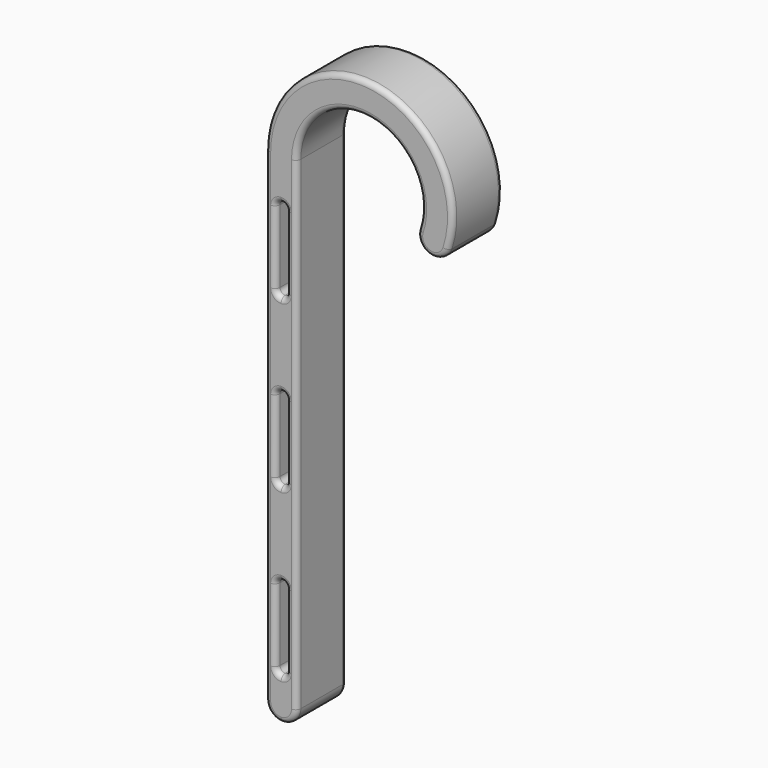
from build123d import *

# Parameters (mm, degrees)
F0_W     = 3.175
F0_H     = 25.4
F1_DEPTH = 19.05
F2_R     = 4.76249
F3_F1_R  = 1.5874
F3_F2_R  = 1.5875
F4_R     = 1.58749


# Not quite as in the source:
# - a fillet or chamfer is up to 0.001 mm smaller than in the source, because OpenCascade refuses the exact size
# - a feature names something its author has since deleted; it is built from what else it names


with BuildPart() as f1:
    # F0 (on Front) → F1 (new body)
    with BuildSketch(Plane.XZ):
        with BuildLine():
            ThreePointArc((17.145, 0), (-11.43, 28.575), (-40.005, 0))
            Line((-40.005, 0), (-40.005, -152.4))
            Line((-40.005, -152.4), (-30.48, -152.4))
            Line((-30.48, -152.4), (-30.48, 0))
            ThreePointArc((-30.48, 0), (-6.4994971908, 18.4008869908), (5.0677839421, -9.525))
            Line((5.0677839421, -9.525), (13.3166759131, -14.2875))
            ThreePointArc((13.3166759131, -14.2875), (16.1713304862, -7.3957542138), (17.145, 0))
        make_face()
        with Locations((-35.2425, -127)):
            Rectangle(F0_W, F0_H, mode=Mode.SUBTRACT)
        with Locations((-35.2425, -76.2)):
            Rectangle(F0_W, F0_H, mode=Mode.SUBTRACT)
        with Locations((-35.2425, -25.4)):
            Rectangle(F0_W, F0_H, mode=Mode.SUBTRACT)
    extrude(amount=F1_DEPTH)

    # F2 (radius 4.7625 in the source; OpenCascade refuses exactly that, so slightly less here)
    f2_edges = [f1.edges().sort_by_distance(p)[0] for p in [
        (13.316676, -9.525, -14.2875),
        (5.067784, -9.525, -9.525),
        (-30.48, -9.525, -152.4),
        (-40.005, -9.525, -152.4),
    ]]
    fillet(f2_edges, radius=F2_R)

    # F3: fillet of radius 1.5875 on 24 edges, made by hand

    # F3_f1 (radius 1.5875 in the source; OpenCascade refuses exactly that, so slightly less here)
    f3_f1_edges = [f1.edges().sort_by_distance(p)[0] for p in [
        (-36.83, -9.525, -12.7),
        (-33.655, -9.525, -12.7),
        (-36.83, -9.525, -63.5),
        (-33.655, -9.525, -63.5),
        (-36.83, -9.525, -114.3),
        (-33.655, -9.525, -114.3),
        (-33.655, -9.525, -139.7),
        (-36.83, -9.525, -139.7),
        (-33.655, -9.525, -88.9),
        (-36.83, -9.525, -88.9),
        (-33.655, -9.525, -38.1),
        (-36.83, -9.525, -38.1),
    ]]
    fillet(f3_f1_edges, radius=F3_F1_R)

    # F3_f2
    f3_f2_edges = [f1.edges().sort_by_distance(p)[0] for p in [
        (-35.2425, 0, -12.7),
        (-35.2425, -19.05, -12.7),
        (-35.2425, 0, -63.5),
        (-35.2425, -19.05, -63.5),
        (-35.2425, 0, -114.3),
        (-35.2425, -19.05, -114.3),
        (-35.2425, 0, -139.7),
        (-35.2425, -19.05, -139.7),
        (-35.2425, 0, -88.9),
        (-35.2425, -19.05, -88.9),
        (-35.2425, 0, -38.1),
        (-35.2425, -19.05, -38.1),
        (-34.1199386955, -19.05, -37.6350613045),
        (-36.3650613045, -19.05, -37.6350613045),
        (-34.1199386955, 0, -37.6350613045),
        (-36.3650613045, 0, -37.6350613045),
        (-34.1199386955, -19.05, -88.4350613045),
        (-36.3650613045, -19.05, -88.4350613045),
        (-34.1199386955, 0, -88.4350613045),
        (-36.3650613045, 0, -88.4350613045),
        (-34.1199386955, -19.05, -139.2350613045),
        (-36.3650613045, -19.05, -139.2350613045),
        (-34.1199386955, 0, -139.2350613045),
        (-36.3650613045, 0, -139.2350613045),
        (-36.3650613045, -19.05, -114.7649386955),
        (-34.1199386955, -19.05, -114.7649386955),
        (-36.3650613045, 0, -114.7649386955),
        (-34.1199386955, 0, -114.7649386955),
        (-36.3650613045, -19.05, -63.9649386955),
        (-34.1199386955, -19.05, -63.9649386955),
        (-36.3650613045, 0, -63.9649386955),
        (-34.1199386955, 0, -63.9649386955),
        (-36.3650613045, -19.05, -13.1649386955),
        (-34.1199386955, -19.05, -13.1649386955),
        (-36.3650613045, 0, -13.1649386955),
        (-34.1199386955, 0, -13.1649386955),
    ]]
    fillet(f3_f2_edges, radius=F3_F2_R)

    # F4 (radius 1.5875 in the source; OpenCascade refuses exactly that, so slightly less here)
    f4_edges = [f1.edges().sort_by_distance(p)[0] for p in [
        (-35.2425, -19.05, -11.1125),
        (-37.487593, -19.05, -12.042407),
        (-32.997407, -19.05, -12.042407),
        (-38.4175, -19.05, -25.4),
        (-32.0675, -19.05, -25.4),
        (-37.487593, -19.05, -38.757593),
        (-32.997407, -19.05, -38.757593),
        (-35.2425, -19.05, -39.6875),
        (-6.845871, -19.05, 28.2049),
        (12.845575, -19.05, -11.994292),
        (-40.005, -19.05, -73.818755),
        (8.775578, -19.05, -11.665696),
        (-38.610099, -19.05, -151.005099),
        (6.703786, -19.05, -9.229997),
        (-35.2425, -19.05, -152.4),
        (-8.373915, -19.05, 18.803267),
        (-31.874901, -19.05, -151.005099),
        (-30.48, -19.05, -73.818755),
        (-35.2425, -19.05, -61.9125),
        (-37.487593, -19.05, -62.842407),
        (-32.997407, -19.05, -62.842407),
        (-38.4175, -19.05, -76.2),
        (-32.0675, -19.05, -76.2),
        (-37.487593, -19.05, -89.557593),
        (-32.997407, -19.05, -89.557593),
        (-35.2425, -19.05, -90.4875),
        (-35.2425, -19.05, -112.7125),
        (-37.487593, -19.05, -113.642407),
        (-32.997407, -19.05, -113.642407),
        (-38.4175, -19.05, -127),
        (-32.0675, -19.05, -127),
        (-37.487593, -19.05, -140.357593),
        (-32.997407, -19.05, -140.357593),
        (-35.2425, -19.05, -141.2875),
        (-35.2425, 0, -11.1125),
        (-37.487593, 0, -12.042407),
        (-32.997407, 0, -12.042407),
        (-38.4175, 0, -25.4),
        (-32.0675, 0, -25.4),
        (-37.487593, 0, -38.757593),
        (-32.997407, 0, -38.757593),
        (-35.2425, 0, -39.6875),
        (-6.845871, 0, 28.2049),
        (12.845575, 0, -11.994292),
        (-40.005, 0, -73.818755),
        (8.775578, 0, -11.665696),
        (-38.610099, 0, -151.005099),
        (6.703786, 0, -9.229997),
        (-35.2425, 0, -152.4),
        (-8.373915, 0, 18.803267),
        (-31.874901, 0, -151.005099),
        (-30.48, 0, -73.818755),
        (-35.2425, 0, -61.9125),
        (-37.487593, 0, -62.842407),
        (-32.997407, 0, -62.842407),
        (-38.4175, 0, -76.2),
        (-32.0675, 0, -76.2),
        (-37.487593, 0, -89.557593),
        (-32.997407, 0, -89.557593),
        (-35.2425, 0, -90.4875),
        (-35.2425, 0, -112.7125),
        (-37.487593, 0, -113.642407),
        (-32.997407, 0, -113.642407),
        (-38.4175, 0, -127),
        (-32.0675, 0, -127),
        (-37.487593, 0, -140.357593),
        (-32.997407, 0, -140.357593),
        (-35.2425, 0, -141.2875),
    ]]
    fillet(f4_edges, radius=F4_R)


solid = f1.part
